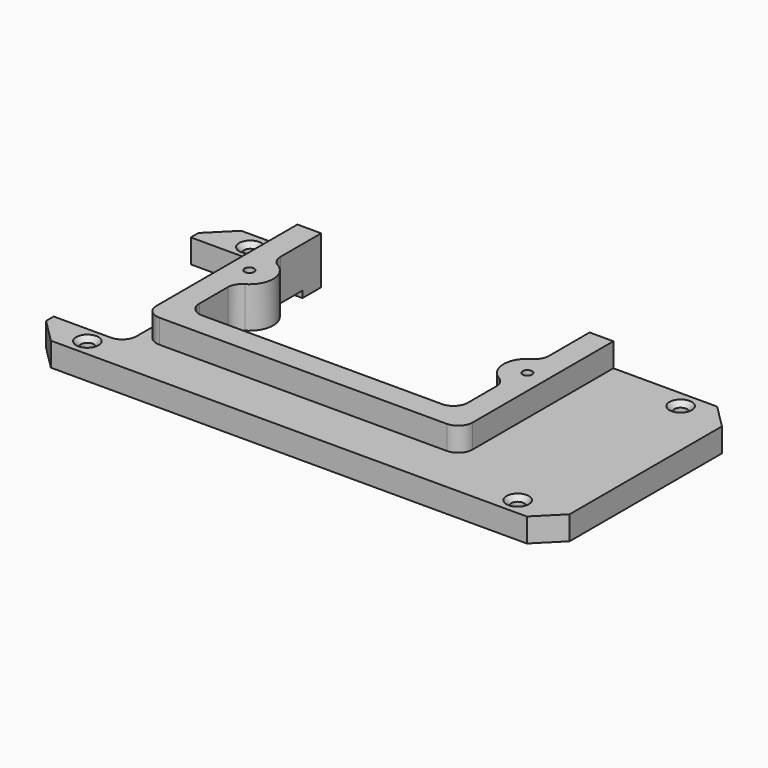
from build123d import *

# Parameters (mm, degrees)
F0_R     = 1.7145
F0_R_2   = 1.27
F1_DEPTH = 6.35
F2_W     = 120.65
F2_H     = 51.054
F3_DEPTH = 1.778
F4_R     = 1.27
F5_DEPTH = 6.35
F6_SIZE  = 6.35
F7_R     = 3.81
F8_SIZE  = 1.27


# Not quite as in the source:
# - a feature names something its author has since deleted; it is built from what else it names


with BuildPart() as f1:
    # F0 (on Top) → F1 (new body)
    with BuildSketch(Plane.XY):
        with BuildLine():
            Line((69.85, -31.75), (69.85, 31.75))
            Line((69.85, 31.75), (29.464, 31.75))
            Line((29.464, 31.75), (29.464, 15.6197039467))
            ThreePointArc((29.464, 15.6197039467), (24.384, 9.398), (29.464, 3.1762960533))
            Line((29.464, 3.1762960533), (29.464, -12.7))
            Line((29.464, -12.7), (-42.164, -12.7))
            Line((-42.164, -12.7), (-42.164, 3.1762960533))
            ThreePointArc((-42.164, 3.1762960533), (-37.084, 9.398), (-42.164, 15.6197039467))
            Line((-42.164, 15.6197039467), (-42.164, 31.75))
            Line((-42.164, 31.75), (-69.85, 31.75))
            Line((-69.85, 31.75), (-69.85, 22.86))
            Line((-69.85, 22.86), (-50.8, 22.86))
            Line((-50.8, 22.86), (-50.8, -22.86))
            Line((-50.8, -22.86), (-69.85, -22.86))
            Line((-69.85, -22.86), (-69.85, -31.75))
            Line((-69.85, -31.75), (69.85, -31.75))
        make_face()
        with Locations((-57.404, -27.178)):
            Circle(F0_R, mode=Mode.SUBTRACT)
        with Locations((57.404, -27.178)):
            Circle(F0_R, mode=Mode.SUBTRACT)
        with Locations((-43.434, 9.398)):
            Circle(F0_R_2, mode=Mode.SUBTRACT)
        with Locations((-57.404, 27.178)):
            Circle(F0_R, mode=Mode.SUBTRACT)
        with Locations((30.734, 9.398)):
            Circle(F0_R_2, mode=Mode.SUBTRACT)
        with Locations((57.404, 27.178)):
            Circle(F0_R, mode=Mode.SUBTRACT)
    extrude(amount=F1_DEPTH)

    # F2 (on Top) → F3 (cut)
    with BuildSketch(Plane.XY):
        Rectangle(F2_W, F2_H)
    extrude(amount=F3_DEPTH, mode=Mode.SUBTRACT)

    # F4 (on face) → F5 (join)
    with BuildSketch(Plane.XY.offset(6.35)):
        with BuildLine():
            Line((-48.514, 31.75), (-48.514, -19.05))
            Line((-48.514, -19.05), (35.814, -19.05))
            Line((35.814, -19.05), (35.814, 31.75))
            Line((35.814, 31.75), (29.464, 31.75))
            Line((29.464, 31.75), (29.464, 15.6197039467))
            ThreePointArc((29.464, 15.6197039467), (24.384, 9.398), (29.464, 3.1762960533))
            Line((29.464, 3.1762960533), (29.464, -12.7))
            Line((29.464, -12.7), (-42.164, -12.7))
            Line((-42.164, -12.7), (-42.164, 3.1762960533))
            ThreePointArc((-42.164, 3.1762960533), (-37.084, 9.398), (-42.164, 15.6197039467))
            Line((-42.164, 15.6197039467), (-42.164, 31.75))
            Line((-42.164, 31.75), (-48.514, 31.75))
        make_face()
        with Locations((-43.434, 9.398)):
            Circle(F4_R, mode=Mode.SUBTRACT)
        with Locations((30.734, 9.398)):
            Circle(F4_R, mode=Mode.SUBTRACT)
    extrude(amount=F5_DEPTH)

    # F6
    f6_edges = [f1.edges().sort_by_distance(p)[0] for p in [
        (-69.85, 31.75, 3.175),
        (69.85, 31.75, 3.175),
        (69.85, -31.75, 3.175),
        (-69.85, -31.75, 3.175),
    ]]
    chamfer(f6_edges, length=F6_SIZE)

    # F7
    f7_edges = [f1.edges().sort_by_distance(p)[0] for p in [
        (-50.8, 22.86, 4.064),
        (-50.8, -22.86, 4.064),
        (29.464, -12.7, 7.239),
        (-42.164, -12.7, 7.239),
        (29.464, 3.176296, 7.239),
        (29.464, 15.619704, 7.239),
        (-42.164, 15.619704, 7.239),
        (-42.164, 3.176296, 7.239),
        (-48.514, -19.05, 9.525),
        (35.814, -19.05, 9.525),
    ]]
    fillet(f7_edges, radius=F7_R)

    # F8
    f8_edges = [f1.edges().sort_by_distance(p)[0] for p in [
        (-59.1185, -27.178, 6.35),
        (-59.1185, 27.178, 6.35),
        (55.6895, 27.178, 6.35),
        (55.6895, -27.178, 6.35),
    ]]
    chamfer(f8_edges, length=F8_SIZE)


solid = f1.part
